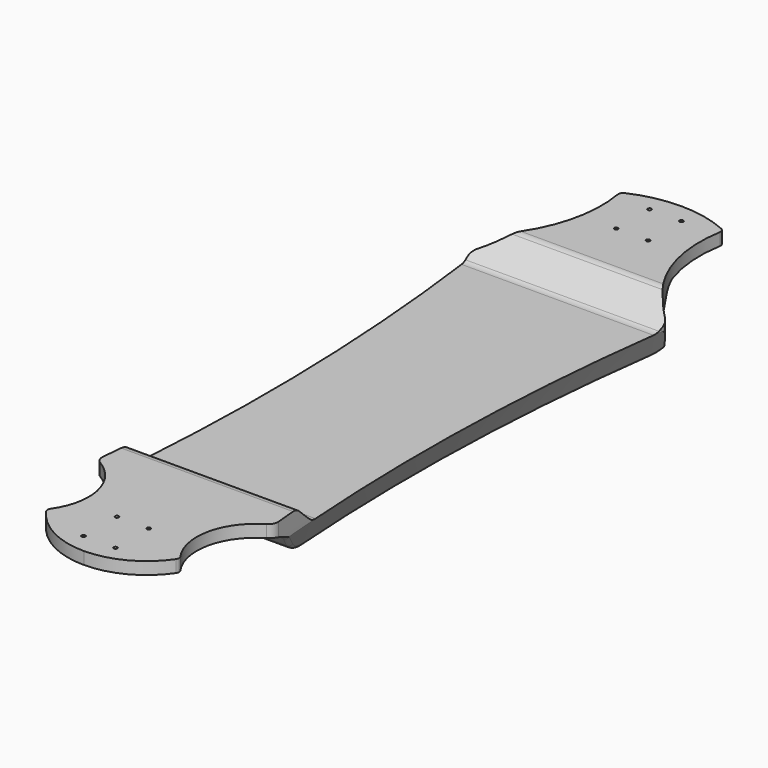
from build123d import *

# Parameters (mm, degrees)
F2_DEPTH    = 28.575
F4_DEPTH    = 125.5709966587
F6_R        = 2.38125
F7_DEPTH    = 28.5760001
F8_T2_ANGLE = 15.450429955
F8_T4_ANGLE = 15.450429955
F9_R        = 5.08


# Not quite as in the source:
# - a fillet or chamfer that OpenCascade refuses, or shapes differently, is made with other operations: its cross-section is extruded or revolved along the edge and cut away or added


with BuildPart() as f2:
    # F1 (on Top) → F2 (new body, symmetric)
    with BuildSketch(Plane.XY):
        with BuildLine():
            ThreePointArc((62.3500417324, 469.2619728609), (31.8803649289, 479.2281930777), (0, 482.6))
            Line((0, 482.6), (0, -482.6))
            ThreePointArc((0, -482.6), (47.3507644076, -470.8914073203), (83.7879301238, -438.4642738192))
            ThreePointArc((83.7879301238, -438.4642738192), (84.9010646272, -434.8337405991), (83.7434010687, -431.2171600359))
            ThreePointArc((83.7434010687, -431.2171600359), (71.5543018167, -371.3240537818), (107.2943853504, -321.7417510283))
            ThreePointArc((107.2943853504, -321.7417510283), (112.1517776655, -316.5709976049), (113.4777772572, -309.601587576))
            ThreePointArc((113.4777772572, -309.601587576), (102.1184741421, -7.6636027846), (125.4548393993, 293.5854544484))
            ThreePointArc((125.4548393993, 293.5854544484), (124.7752527295, 299.7139243562), (121.2893072339, 304.8))
            ThreePointArc((121.2893072339, 304.8), (73.165621714, 376.4071058547), (66.0091903509, 462.3853135997))
            ThreePointArc((66.0091903509, 462.3853135997), (65.3579062685, 466.4506248637), (62.3500417324, 469.2619728609))
        make_face()
    extrude(amount=F2_DEPTH, both=True)

    # F3 (on Right) → F4 (cut, through all)
    with BuildSketch(Plane.YZ):
        with BuildLine():
            ThreePointArc((330.9678458452, 26.7136872014), (334.5828269011, 28.1026444048), (338.4265451971, 28.575))
            Line((338.4265451971, 28.575), (-283.4437722547, 28.575))
            ThreePointArc((-283.4437722547, 28.575), (-277.71711362, 27.5061138008), (-272.7616230334, 24.4433944417))
            Line((-272.7616230334, 24.4433944417), (-253.9223363738, 7.3066055583))
            ThreePointArc((-253.9223363738, 7.3066055583), (-248.9668457872, 4.2438861992), (-243.2401871524, 3.175))
            Line((-243.2401871524, 3.175), (282.7808733864, 3.175))
            ThreePointArc((282.7808733864, 3.175), (286.6245916824, 3.6473555952), (290.2395727383, 5.0363127986))
            Line((290.2395727383, 5.0363127986), (330.9678458452, 26.7136872014))
        make_face()
        with BuildLine():
            Line((482.6, -28.575), (482.6, 12.7))
            Line((482.6, 12.7), (379.5943665901, 12.7))
            ThreePointArc((379.5943665901, 12.7), (368.7657733725, 11.1287772712), (358.8303104324, 6.5447017811))
            Line((358.8303104324, 6.5447017811), (314.2696895676, -22.4197017811))
            ThreePointArc((314.2696895676, -22.4197017811), (304.3342266275, -27.0037772712), (293.5056334099, -28.575))
            Line((293.5056334099, -28.575), (482.6, -28.575))
        make_face()
        with BuildLine():
            Line((-321.4813699303, 12.7), (-482.6, 12.7))
            Line((-482.6, 12.7), (-482.6, -28.575))
            Line((-482.6, -28.575), (-250.0186300697, -28.575))
            ThreePointArc((-250.0186300697, -28.575), (-265.2995302407, -25.3763479677), (-278.01464131, -16.3174719141))
            Line((-278.01464131, -16.3174719141), (-293.48535869, 0.4424719141))
            ThreePointArc((-293.48535869, 0.4424719141), (-306.2004697593, 9.5013479677), (-321.4813699303, 12.7))
        make_face()
    extrude(amount=F4_DEPTH, mode=Mode.SUBTRACT)

    # F5: F2 across plane


with BuildPart() as f2_1:
    add(f2.part)
    add(f2.part.mirror(Plane.YZ))

    # F6 (on Top) → F7 (cut, through all)
    with BuildSketch(Plane.XY):
        with Locations((-20.6375, 403.225)):
            Circle(F6_R)
        with Locations((20.6375, 403.225)):
            Circle(F6_R)
        with Locations((20.6375, 457.2)):
            Circle(F6_R)
        with Locations((-20.6375, 457.2)):
            Circle(F6_R)
        with Locations((-20.6375, -457.2)):
            Circle(F6_R)
        with Locations((20.6375, -457.2)):
            Circle(F6_R)
        with Locations((20.6375, -403.225)):
            Circle(F6_R)
        with Locations((-20.6375, -403.225)):
            Circle(F6_R)
    extrude(amount=F7_DEPTH, mode=Mode.SUBTRACT)

    # F8: chamfer of 12.7 x 31.75 on 2 edges, made by hand

    # F8_s1 → F8_t2 (revolve, cut)
    with BuildSketch(Plane(origin=(35.3998327569, -340.3813995604, 0), x_dir=(0, 0, 1), z_dir=(0.1034425731, -0.9946354277, 0))):
        Polygon((3.175, -80.7464889634), (-28.575, -68.0464889634), (-28.575, -80.7464889634), align=None)
    revolve(axis=Axis((2732.4064480743, -59.8913867398, -28.575), (0, 0, -1)), revolution_arc=F8_T2_ANGLE, mode=Mode.SUBTRACT)

    # F8_s3 → F8_t4 (revolve, cut)
    with BuildSketch(Plane(origin=(-35.3998327569, -340.3813995604, 0), x_dir=(0, 0, 1), z_dir=(-0.1034425731, -0.9946354277, 0))):
        Polygon((3.175, 80.7464889634), (-28.575, 68.0464889634), (-28.575, 80.7464889634), align=None)
    revolve(axis=Axis((-2732.4064480743, -59.8913867398, -28.575), (0, 0, 1)), revolution_arc=F8_T4_ANGLE, mode=Mode.SUBTRACT)

    # F9
    f9_edges = [f2_1.edges().sort_by_distance(p)[0] for p in [
        (-90.17428, 22.178757, -28.575),
        (90.17428, 22.178757, -28.575),
        (-114.168649, 301.970074, -27.622857),
        (114.168649, 301.970074, -27.622857),
        (111.571684, -294.833445, 1.830462),
        (106.854727, -285.755936, -7.931069),
        (98.500194, -266.535273, -24.80881),
        (-111.571684, -294.833445, 1.830462),
        (-106.854727, -285.755936, -7.931069),
        (-98.500194, -266.535273, -24.80881),
    ]]
    fillet(f9_edges, radius=F9_R)


solid = f2_1.part
